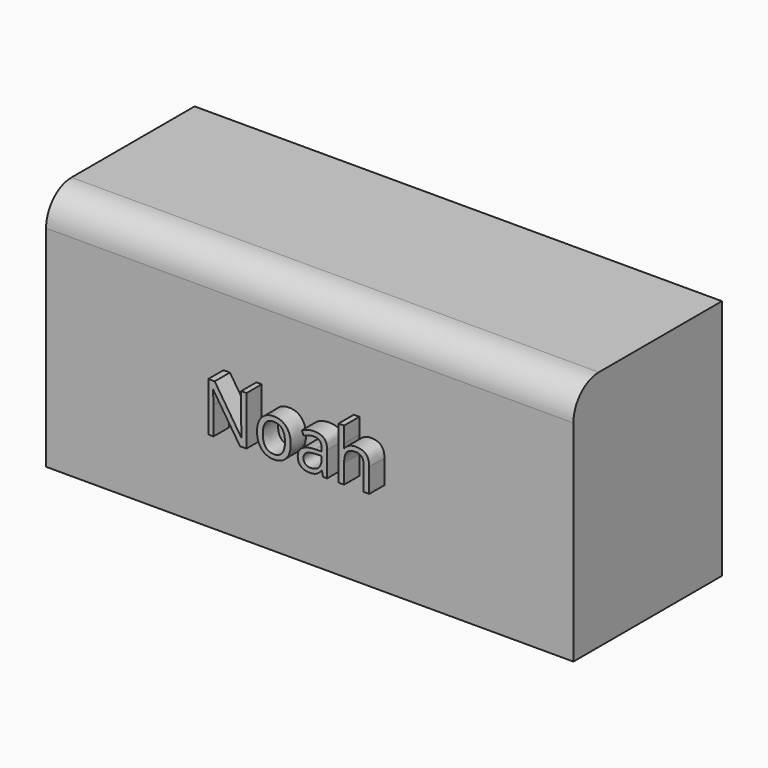
from build123d import *

# Parameters (mm, degrees)
F0_W         = 84.4128280878
F0_H         = 38.7145169079
F1_DEPTH     = 29.718
F2_T         = -2.54
F3_R         = 5.08
F4_TEXT_SIZE = 10.9648978752
F5_DEPTH     = 32.766


# Not quite as in the source:
# - Text() gives the source's letters only with a copy of the font that has no kerning and outlines rounded to 1/6400 em; it was checked with that copy


with BuildPart() as f1:
    # F0 (on Front) → F1 (new body)
    with BuildSketch(Plane.XZ):
        with Locations((1.821860671, 19.357258454)):
            Rectangle(F0_W, F0_H)
    extrude(amount=F1_DEPTH)

    # F2
    f2_openings = [f1.faces().sort_by_distance(p)[0] for p in [
        (1.821861, -14.859, 0),
    ]]
    offset(amount=F2_T, openings=f2_openings)

    # F3
    f3_edges = [f1.edges().sort_by_distance(p)[0] for p in [
        (1.821861, -29.718, 38.714517),
    ]]
    fillet(f3_edges, radius=F3_R)

    # F4 (on Front) → F5 (join)
    with BuildSketch(Plane.XZ):
        with Locations((-13.0566619337, 15.0303412229)):
            Text('Noah', F4_TEXT_SIZE, font='Open Sans', text_align=(TextAlign.LEFT, TextAlign.BOTTOM))
    extrude(amount=F5_DEPTH)


solid = f1.part
